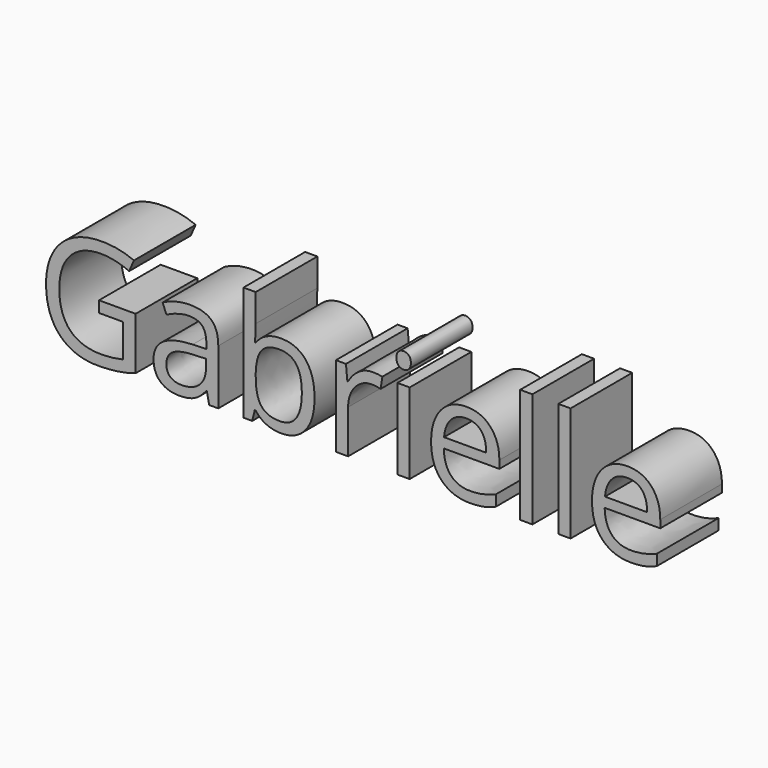
from build123d import *

# Parameters (mm, degrees)
F0_TEXT_SIZE = 48.2006076102
F1_DEPTH     = 24.638


# Not quite as in the source:
# - Text() gives the source's letters only with a copy of the font that has no kerning and outlines rounded to 1/6400 em; it was checked with that copy


with BuildPart() as f1:
    # F0 (on Front) → F1 (new body)
    with BuildSketch(Plane.XZ):
        with Locations((-150.6926864386, -17.6050942391)):
            Text('Gabrielle', F0_TEXT_SIZE, font='Open Sans', text_align=(TextAlign.LEFT, TextAlign.BOTTOM))
    extrude(amount=F1_DEPTH)


solid = f1.part
